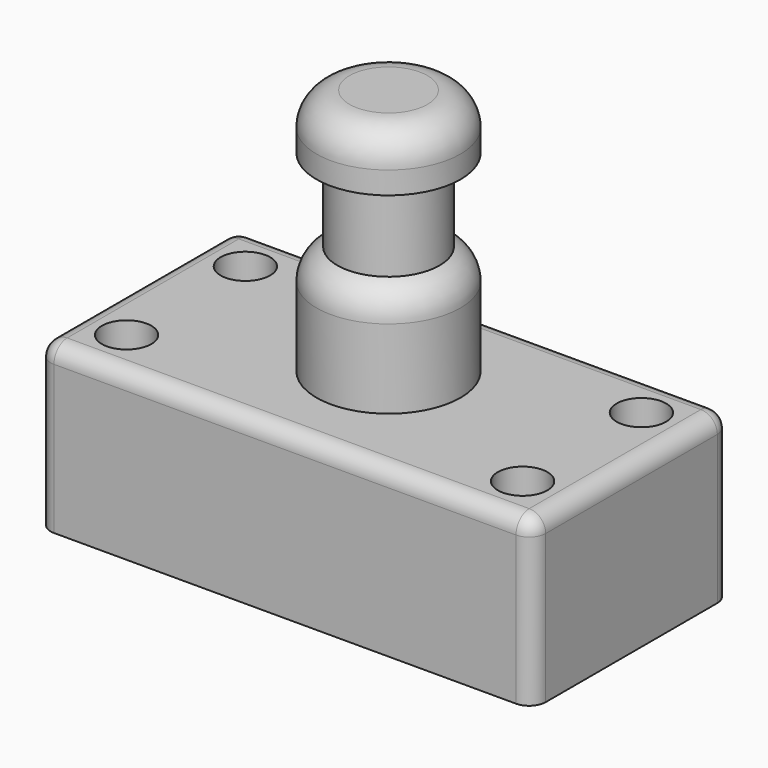
from build123d import *

# Parameters (mm, degrees)
F0_W          = 76.2
F0_H          = 38.1
F1_DEPTH      = 25.4
F3_R          = 3.81
F4_DEPTH      = 25.4
F5_R          = 11.0802185983
F6_DEPTH      = 38.1
F2_R          = 3.81
F7_DEPTH      = 25.4
F8_R          = 3.81
F9_DEPTH      = 25.4
F11_R         = 3.81
F12_DEPTH     = 25.4
F10_W         = 12.7
F10_H         = 12.7
F14_R         = 2.54
F15_R         = 2.54
F17_T1_DEPTH  = 29.21
F17_S5_W      = 2.54
F17_S5_H      = 2.54
F17_T6_DEPTH  = 2.54
F17_S11_W     = 2.54
F17_S11_H     = 2.54
F17_T12_DEPTH = 2.54


# Not quite as in the source:
# - a fillet or chamfer that OpenCascade refuses, or shapes differently, is made with other operations: its cross-section is extruded or revolved along the edge and cut away or added


with BuildPart() as f1:
    # F0 (on Top) → F1 (new body)
    with BuildSketch(Plane.XY):
        with Locations((2.4286340922, -4.9461158044)):
            Rectangle(F0_W, F0_H)
    extrude(amount=F1_DEPTH)

    # F3 (on face) → F4 (cut)
    with BuildSketch(Plane.XY.offset(25.4)):
        with Locations((32.9086340922, 6.4838841956)):
            Circle(F3_R)
    extrude(amount=-F4_DEPTH, mode=Mode.SUBTRACT)

    # F5 (on face) → F6 (join)
    with BuildSketch(Plane.XY.offset(25.4)):
        with Locations((2.4286331609, -4.0792874061)):
            Circle(F5_R)
    extrude(amount=F6_DEPTH)

    # F2 (on face) → F7 (cut)
    with BuildSketch(Plane.XY.offset(25.4)):
        with Locations((-28.0513659078, 6.4838841956)):
            Circle(F2_R)
    extrude(amount=-F7_DEPTH, mode=Mode.SUBTRACT)

    # F8 (on face) → F9 (cut)
    with BuildSketch(Plane.XY.offset(25.4)):
        with Locations((-28.0513659078, -16.3761158044)):
            Circle(F8_R)
    extrude(amount=-F9_DEPTH, mode=Mode.SUBTRACT)

    # F11 (on face) → F12 (cut)
    with BuildSketch(Plane.XY.offset(25.4)):
        with Locations((32.9086340922, -16.3761158044)):
            Circle(F11_R)
    extrude(amount=-F12_DEPTH, mode=Mode.SUBTRACT)

    # F10 (on Front) → F13 (revolve, cut)
    with BuildSketch(Plane.XZ):
        with Locations((-10.6504372485, 48.6334538215)):
            Rectangle(F10_W, F10_H)
    revolve(axis=Axis((2.4286331609, -4.0792874061, 25.4), (0, 0, -1)), mode=Mode.SUBTRACT)

    # F14
    f14_edges = [f1.edges().sort_by_distance(p)[0] for p in [
        (2.428634, -23.996116, 25.4),
    ]]
    fillet(f14_edges, radius=F14_R)

    # F15
    f15_edges = [f1.edges().sort_by_distance(p)[0] for p in [
        (-35.671366, -3.676116, 25.4),
        (2.428634, 14.103884, 25.4),
        (40.528634, -3.676116, 25.4),
    ]]
    fillet(f15_edges, radius=F15_R)

    # F16: fillet of radius 5.08 on 2 edges, made by hand

    # F16_s1 → F16_t2 (revolve, cut)
    with BuildSketch(Plane.XZ.offset(4.0792874061)):
        with BuildLine():
            ThreePointArc((13.5088517592, 58.42), (12.0209542077, 62.0121024484), (8.4288517592, 63.5))
            Line((8.4288517592, 63.5), (8.4288517592, 63.6016))
            Line((8.4288517592, 63.6016), (13.6104517592, 63.6016))
            Line((13.6104517592, 63.6016), (13.6104517592, 58.42))
            Line((13.6104517592, 58.42), (13.5088517592, 58.42))
        make_face()
    revolve(axis=Axis((2.4286331609, -4.0792874061, 63.5), (0, 0, 1)), mode=Mode.SUBTRACT)

    # F16_s3 → F16_t4 (revolve, cut)
    with BuildSketch(Plane.XZ.offset(4.0792874061)):
        with BuildLine():
            ThreePointArc((13.5088517592, 37.5596735125), (12.630027146, 40.4156366371), (10.2976212989, 42.2834538215))
            Line((10.2976212989, 42.2834538215), (10.3349966897, 42.3779294277))
            ThreePointArc((10.3349966897, 42.3779294277), (11.9032365291, 42.3850538215), (13.5088517592, 42.3850538215))
            Line((13.5088517592, 42.3850538215), (13.6104517592, 42.2834538215))
            Line((13.6104517592, 42.2834538215), (13.6104517592, 37.5596735125))
            Line((13.6104517592, 37.5596735125), (13.5088517592, 37.5596735125))
        make_face()
    revolve(axis=Axis((2.4286331609, -4.0792874061, 42.2834538215), (0, 0, -1)), mode=Mode.SUBTRACT)

    # F17: fillet of radius 2.54 on 2 edges, made by hand

    # F17_s2 → F17_t1 (cut)
    with BuildSketch(Plane.XY.offset(-6.35)):
        with BuildLine():
            ThreePointArc((-35.6713659078, 11.5638841956), (-34.927417132, 13.3599354199), (-33.1313659078, 14.1038841956))
            Line((-33.1313659078, 14.1038841956), (-35.6713659078, 14.1038841956))
            Line((-35.6713659078, 14.1038841956), (-35.6713659078, 11.5638841956))
        make_face()
        with BuildLine():
            ThreePointArc((40.5286340922, 11.5638841956), (39.7846853164, 13.3599354199), (37.9886340922, 14.1038841956))
            Line((37.9886340922, 14.1038841956), (40.5286340922, 14.1038841956))
            Line((40.5286340922, 14.1038841956), (40.5286340922, 11.5638841956))
        make_face()
    extrude(amount=F17_T1_DEPTH, mode=Mode.SUBTRACT)


with BuildPart() as f17_tool4:
    # F17_s5 → F17_t6 (new body)
    with BuildSketch(Plane.YZ.offset(37.9886340922)):
        with Locations((12.8338841956, 24.13)):
            Rectangle(F17_S5_W, F17_S5_H)
    extrude(amount=F17_T6_DEPTH)

    # F17_s7 → F17_t8 (revolve, cut)
    with BuildSketch(Plane(origin=(37.9886340922, 11.5638841956, 22.86), x_dir=(0, -0.7071067812, -0.7071067812), z_dir=(0, -0.7071067812, 0.7071067812))):
        with BuildLine():
            ThreePointArc((0, -2.54), (2.54, 0), (0, 2.54))
            Line((0, 2.54), (0, -2.54))
        make_face()
    revolve(axis=Axis((37.9886340922, 11.5638841956, 22.86), (1, 0, 0)), mode=Mode.SUBTRACT)


with BuildPart() as f1_1:
    add(f1.part)

    # F17_t3: cut F17_tool4
    add(f17_tool4.part, mode=Mode.SUBTRACT)


with BuildPart() as f17_tool10:
    # F17_s11 → F17_t12 (new body)
    with BuildSketch(Plane.YZ.offset(-33.1313659078)):
        with Locations((12.8338841956, 24.13)):
            Rectangle(F17_S11_W, F17_S11_H)
    extrude(amount=-F17_T12_DEPTH)

    # F17_s13 → F17_t14 (revolve, cut)
    with BuildSketch(Plane(origin=(-33.1313659078, 11.5638841956, 22.86), x_dir=(0, -0.7071067812, -0.7071067812), z_dir=(0, 0.7071067812, -0.7071067812))):
        with BuildLine():
            ThreePointArc((0, -2.54), (2.54, 0), (0, 2.54))
            Line((0, 2.54), (0, -2.54))
        make_face()
    revolve(axis=Axis((-33.1313659078, 11.5638841956, 22.86), (-1, 0, 0)), mode=Mode.SUBTRACT)


with BuildPart() as f1_2:
    add(f1_1.part)

    # F17_t9: cut F17_tool10
    add(f17_tool10.part, mode=Mode.SUBTRACT)


solid = f1_2.part
